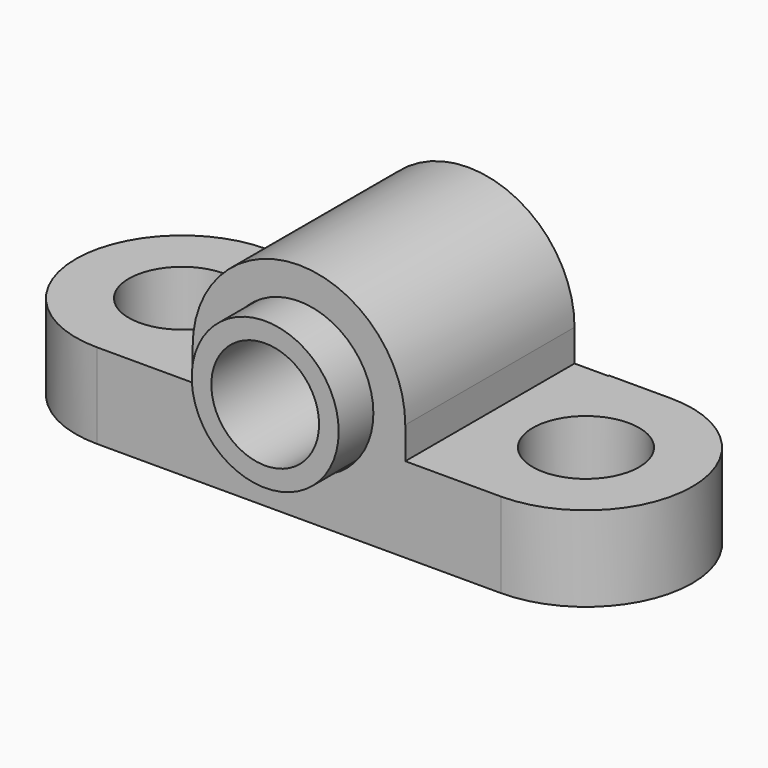
from build123d import *

# Parameters (mm, degrees)
F0_R      = 5.0038
F1_DEPTH  = 8
F3_R      = 7
F4_DEPTH  = 10.001
F5_DEPTH  = 25.4
F2_R      = 7
F6_DEPTH  = 20.0152
F7_DEPTH  = 4
F8_R      = 6.9149317759
F8_R_2    = 5.0676799546
F9_DEPTH  = 13.97127
F11_W     = 24.9205389991
F11_H     = 28.2232568134
F12_DEPTH = 25.4


# Not quite as in the source:
# - a feature of the source that left no trace in its solid (it failed there, or was rolled back) is left out


with BuildPart() as f1:
    # F0 (on Top) → F1 (new body)
    with BuildSketch(Plane.XY):
        with BuildLine():
            ThreePointArc((-19, 10), (-29, 0), (-19, -10))
            Line((-19, -10), (19, -10))
            ThreePointArc((19, -10), (29, 0), (19, 10))
            Line((19, 10), (-19, 10))
        make_face()
        with Locations((-19, 0)):
            Circle(F0_R, mode=Mode.SUBTRACT)
        with Locations((19, 0)):
            Circle(F0_R, mode=Mode.SUBTRACT)
    extrude(amount=F1_DEPTH)

    # F3 (on Front) → F4 (cut, through all)
    with BuildSketch(Plane.XZ):
        with Locations((0, 11)):
            Circle(F3_R)
    extrude(amount=-F4_DEPTH, mode=Mode.SUBTRACT)

    # F5 (cut): a face of the model
    f5_faces = [f1.faces().sort_by_distance(p)[0] for p in [
        (0, 0, 6.3529291392),
    ]]
    extrude(f5_faces, amount=-F5_DEPTH, mode=Mode.SUBTRACT)

    # F2 (on face) → F6 (join)
    with BuildSketch(Plane.XZ.offset(10)):
        with BuildLine():
            Line((10, 0), (10, 8))
            Line((10, 8), (10, 11))
            ThreePointArc((10, 11), (0, 21), (-10, 11))
            Line((-10, 11), (-10, 8))
            Line((-10, 8), (-10, 0))
            Line((-10, 0), (10, 0))
        make_face()
        with Locations((0, 11)):
            Circle(F2_R, mode=Mode.SUBTRACT)
    extrude(amount=-F6_DEPTH)

    # F7 (add): a face of the model
    f7_faces = [f1.faces().sort_by_distance(p)[0] for p in [
        (9.71, 10.0152, 5.5),
    ]]
    extrude(f7_faces, amount=F7_DEPTH)


with BuildPart() as f9:
    # F8 (on Front) → F9 (new body, symmetric)
    with BuildSketch(Plane.XZ):
        with Locations((0, 11.0604921356)):
            Circle(F8_R)
        with Locations((0, 11.0604921356)):
            Circle(F8_R_2, mode=Mode.SUBTRACT)
    extrude(amount=F9_DEPTH, both=True)


with BuildPart() as f12_tool:
    # F11 (on offset) → F12 (new body)
    with BuildSketch(Plane.XZ.offset(-9.906)):
        with Locations((0.7121074013, 11.3045781618)):
            Rectangle(F11_W, F11_H)
    extrude(amount=-F12_DEPTH)


with BuildPart() as f1_1:
    add(f1.part)

    # F12: cut by f12_tool
    add(f12_tool.part, mode=Mode.SUBTRACT)


with BuildPart() as f9_1:
    add(f9.part)

    # F12: cut by f12_tool
    add(f12_tool.part, mode=Mode.SUBTRACT)


solid = Compound([f1_1.part, f9_1.part])
